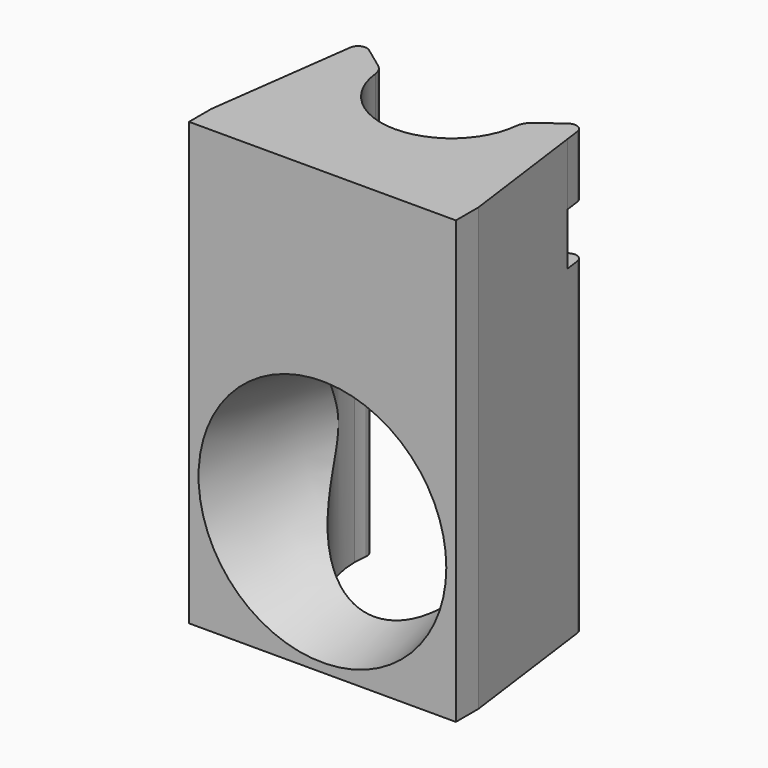
from build123d import *

# Parameters (mm, degrees)
F0_W         = 50.8
F0_H         = 50.8
F1_DEPTH     = 30
F2_W         = 50.8
F2_H         = 50.8
F3_DEPTH     = 30
F5_R         = 10
F4_R         = 14
F8_DEPTH     = 7
F10_DEPTH    = 5.9
F12_DEPTH    = 7
F13_T1_DEPTH = 9.3614920568
F13_T3_DEPTH = 9.3614920568
F14_R        = 1


# Not quite as in the source:
# - a fillet or chamfer that OpenCascade refuses, or shapes differently, is made with other operations: its cross-section is extruded or revolved along the edge and cut away or added


with BuildPart() as f1:
    # F0 (on Top) → F1 (new body)
    with BuildSketch(Plane.XY):
        Rectangle(F0_W, F0_H)
    extrude(amount=F1_DEPTH)

    # F2 (on face) → F3 (cut, through all)
    with BuildSketch(Plane.XY.offset(30)):
        Rectangle(F2_W, F2_H)
        with BuildLine():
            ThreePointArc((-12.8399150562, 1.7135403152), (-11.7164214446, 2.5724711068), (-10.857490653, 1.4489774952))
            ThreePointArc((-10.857490653, 1.4489774952), (-10.9296586704, 0.7260856773), (-10.95375, 0))
            Line((-10.95375, 0), (10.95375, 0))
            ThreePointArc((10.95375, 0), (10.9296586704, 0.7260856773), (10.857490653, 1.4489774952))
            ThreePointArc((10.857490653, 1.4489774952), (11.7164214446, 2.5724711068), (12.8399150562, 1.7135403152))
            Line((12.8399150562, 1.7135403152), (15.08125, -15.08125))
            Line((15.08125, -15.08125), (15.08125, -18.25625))
            Line((15.08125, -18.25625), (-15.08125, -18.25625))
            Line((-15.08125, -18.25625), (-15.08125, -15.08125))
            Line((-15.08125, -15.08125), (-12.8399150562, 1.7135403152))
        make_face(mode=Mode.SUBTRACT)
        with BuildLine():
            Line((10.95375, 0), (-10.95375, 0))
            ThreePointArc((-10.95375, 0), (0, -10.95375), (10.95375, 0))
        make_face()
    extrude(amount=-F3_DEPTH, mode=Mode.SUBTRACT)

    # F5 (on Front) → F6 section 0
    with BuildSketch(Plane.XZ):
        with Locations((0, 15)):
            Circle(F5_R)
    # F4 (on face) → F6 section 1
    with BuildSketch(Plane.XZ.offset(18.25625)):
        with Locations((0, 15)):
            Circle(F4_R)
    loft(mode=Mode.SUBTRACT)

    # F7 (on face) → F8 (join)
    with BuildSketch(Plane.XY.offset(30)):
        with BuildLine():
            ThreePointArc((-10.857490653, 1.4489774952), (-10.9287333274, 1.9732487889), (-11.2575085067, 2.3877880386))
            ThreePointArc((-11.2575085067, 2.3877880386), (-12.2406927383, 2.5012284324), (-12.8399150562, 1.7135403152))
            Line((-12.8399150562, 1.7135403152), (-15.08125, -15.08125))
            Line((-15.08125, -15.08125), (-15.08125, -18.25625))
            Line((-15.08125, -18.25625), (15.08125, -18.25625))
            Line((15.08125, -18.25625), (15.08125, -15.08125))
            Line((15.08125, -15.08125), (12.8399150562, 1.7135403152))
            ThreePointArc((12.8399150562, 1.7135403152), (12.2406927383, 2.5012284324), (11.2575085067, 2.3877880386))
            ThreePointArc((11.2575085067, 2.3877880386), (10.9287333274, 1.9732487889), (10.857490653, 1.4489774952))
            ThreePointArc((10.8574906531, 1.4489774952), (0, -10.95375), (-10.857490653, 1.4489774952))
        make_face()
        with BuildLine():
            ThreePointArc((8, 0), (0, -8), (-8, 0))
            Line((-8, 0), (-11.2575085067, 2.3877880386))
            ThreePointArc((-11.2575085067, 2.3877880386), (-10.9287333274, 1.9732487889), (-10.857490653, 1.4489774952))
            ThreePointArc((-10.857490653, 1.4489774952), (0, -10.95375), (10.8574906531, 1.4489774952))
            ThreePointArc((10.857490653, 1.4489774952), (10.9287333274, 1.9732487889), (11.2575085067, 2.3877880386))
            Line((11.2575085067, 2.3877880386), (8, 0))
        make_face()
    extrude(amount=F8_DEPTH)

    # F9 (on face) → F10 (join)
    with BuildSketch(Plane.XY.offset(37)):
        with BuildLine():
            ThreePointArc((8, 0), (0, -8), (-8, 0))
            Line((-8, 0), (-13.0685941712, 0))
            Line((-13.0685941712, 0), (-15.08125, -15.08125))
            Line((-15.08125, -15.08125), (-15.08125, -18.25625))
            Line((-15.08125, -18.25625), (15.08125, -18.25625))
            Line((15.08125, -18.25625), (15.08125, -15.08125))
            Line((15.08125, -15.08125), (13.0685941712, 0))
            Line((13.0685941712, 0), (8, 0))
        make_face()
        with BuildLine():
            ThreePointArc((6, 0), (0, -6), (-6, 0))
            Line((-6, 0), (-8, 0))
            ThreePointArc((-8, 0), (0, -8), (8, 0))
            Line((8, 0), (6, 0))
        make_face()
    extrude(amount=F10_DEPTH)

    # F11 (on face) → F12 (join)
    with BuildSketch(Plane.XY.offset(42.9)):
        with BuildLine():
            Line((11.2575085067, 2.3877880386), (8, 0))
            Line((8, 0), (13.0685941712, 0))
            Line((13.0685941712, 0), (12.8399150562, 1.7135403152))
            ThreePointArc((12.8399150562, 1.7135403152), (12.2406927383, 2.5012284324), (11.2575085067, 2.3877880386))
        make_face()
        with BuildLine():
            Line((-13.0685941712, 0), (-8, 0))
            Line((-8, 0), (-11.2575085067, 2.3877880386))
            ThreePointArc((-11.2575085067, 2.3877880386), (-12.2406927383, 2.5012284324), (-12.8399150562, 1.7135403152))
            Line((-12.8399150562, 1.7135403152), (-13.0685941712, 0))
        make_face()
        with BuildLine():
            ThreePointArc((8, 0), (0, -8), (-8, 0))
            Line((-8, 0), (-13.0685941712, 0))
            Line((-13.0685941712, 0), (-15.08125, -15.08125))
            Line((-15.08125, -15.08125), (-15.08125, -18.25625))
            Line((-15.08125, -18.25625), (15.08125, -18.25625))
            Line((15.08125, -18.25625), (15.08125, -15.08125))
            Line((15.08125, -15.08125), (13.0685941712, 0))
            Line((13.0685941712, 0), (8, 0))
        make_face()
    extrude(amount=F12_DEPTH)

    # F13: fillet of radius 2 on 4 edges, made by hand

    # F13_s2 → F13_t1 (cut)
    with BuildSketch(Plane.XY.offset(42.9)):
        with BuildLine():
            ThreePointArc((-7.9553868421, -0.8436943713), (-8.2105441596, -0.0574614627), (-8.7618448568, 0.5584403027))
            Line((-8.7618448568, 0.5584403027), (-8, 0))
            ThreePointArc((-8, 0), (-7.9888389249, -0.4224365414), (-7.9553868421, -0.8436943713))
        make_face()
        with BuildLine():
            ThreePointArc((7.9553868421, -0.8436943713), (8.2105441596, -0.0574614627), (8.7618448568, 0.5584403027))
            Line((8.7618448568, 0.5584403027), (8, 0))
            ThreePointArc((8, 0), (7.9888389249, -0.4224365414), (7.9553868421, -0.8436943713))
        make_face()
    extrude(amount=F13_T1_DEPTH, mode=Mode.SUBTRACT)

    # F13_s4 → F13_t3 (cut)
    with BuildSketch(Plane.XY.offset(27.6385079432)):
        with BuildLine():
            ThreePointArc((-7.9553868421, -0.8436943713), (-8.2105441596, -0.0574614627), (-8.7618448568, 0.5584403027))
            Line((-8.7618448568, 0.5584403027), (-8, 0))
            ThreePointArc((-8, 0), (-7.9888389249, -0.4224365414), (-7.9553868421, -0.8436943713))
        make_face()
        with BuildLine():
            ThreePointArc((7.9553868421, -0.8436943713), (8.2105441596, -0.0574614627), (8.7618448568, 0.5584403027))
            Line((8.7618448568, 0.5584403027), (8, 0))
            ThreePointArc((8, 0), (7.9888389249, -0.4224365414), (7.9553868421, -0.8436943713))
        make_face()
    extrude(amount=F13_T3_DEPTH, mode=Mode.SUBTRACT)

    # F14
    f14_edges = [f1.edges().sort_by_distance(p)[0] for p in [
        (-6, 0, 39.95),
        (6, 0, 39.95),
    ]]
    fillet(f14_edges, radius=F14_R)


solid = f1.part
